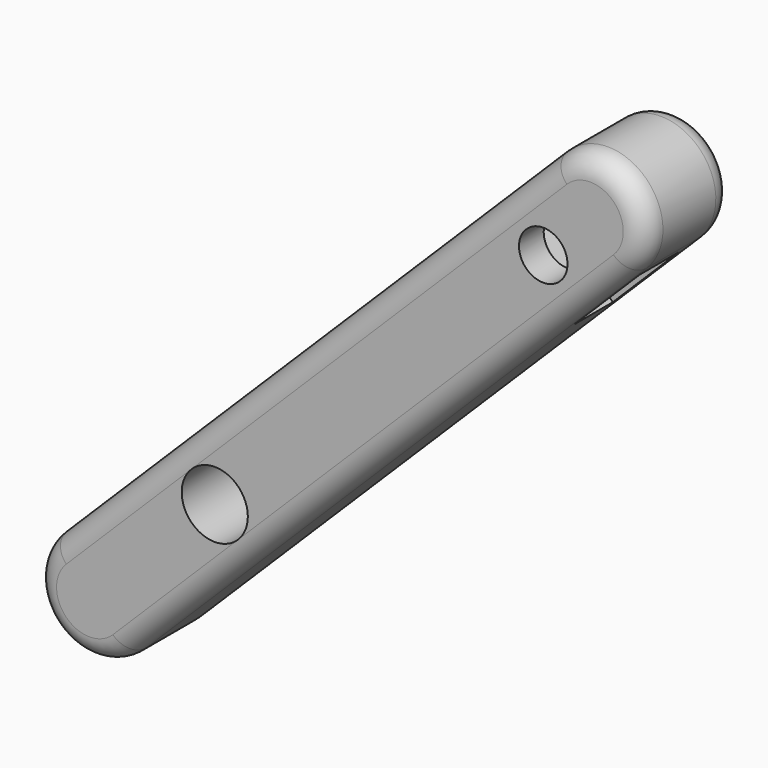
from build123d import *

# Parameters (mm, degrees)
F0_R     = 1.5
F1_DEPTH = 2.5
F2_DEPTH = 5
F3_R     = 0.99999
F6_DEPTH = 1.1
F7_D     = 2.2
F7_DEPTH = 2.501
F8_D     = 2.2


# Not quite as in the source:
# - a fillet or chamfer is up to 0.001 mm smaller than in the source, because OpenCascade refuses the exact size


with BuildPart() as f1:
    # F0 (on Front) → F1 (new body, symmetric)
    with BuildSketch(Plane.XZ):
        with BuildLine():
            ThreePointArc((-7.4377474476, -3.8639245472), (-7.4497190923, -7.3994381845), (-3.9142054549, -7.4114098292))
            Line((-3.9142054549, -7.4114098292), (18.78970035, 15.1392589236))
            ThreePointArc((18.78970035, 15.1392589236), (18.8016719947, 18.6747725609), (15.2661583574, 18.6867442056))
            Line((15.2661583574, 18.6867442056), (-7.4377474476, -3.8639245472))
        make_face()
        Circle(F0_R, mode=Mode.SUBTRACT)
        Circle(F0_R)
    extrude(amount=F1_DEPTH, both=True)

    # F0 (on Front) → F2 (cut, symmetric)
    with BuildSketch(Plane.XZ):
        Circle(F0_R)
    extrude(amount=F2_DEPTH, both=True, mode=Mode.SUBTRACT)

    # F3 (radius 1 in the source; OpenCascade refuses exactly that, so slightly less here)
    f3_edges = [f1.edges().sort_by_distance(p)[0] for p in [
        (3.914205, -2.5, 7.41141),
        (3.914205, 2.5, 7.41141),
    ]]
    fillet(f3_edges, radius=F3_R)

    # F5 (on Front) → F6 (cut, symmetric)
    with BuildSketch(Plane.XZ):
        Polygon((17.2437955285, 15.4185445413), (16.6082652356, 13.0784374397), (14.2639078916, 12.4587692675), (15.1712653624, 11.5452460911), (18.1511529993, 14.5050213649), align=None)
        Polygon((14.2639078916, 12.4587692675), (16.6082652356, 13.0784374397), (17.2437955285, 15.4185445413), (15.5349684774, 17.1389834706), (13.1906111334, 16.5193152984), (12.5550808405, 14.1792081968), align=None)
        Polygon((11.6477233698, 15.0927313731), (12.5550808405, 14.1792081968), (13.1906111334, 16.5193152984), (15.5349684774, 17.1389834706), (14.6276110067, 18.0525066469), align=None)
    extrude(amount=F6_DEPTH, both=True, mode=Mode.SUBTRACT)

    # F7 (through all, one way)
    with BuildSketch(Plane.XZ):
        with Locations((14.8994381845, 14.798876369)):
            Circle(F7_D / 2)
    extrude(amount=-F7_DEPTH, mode=Mode.SUBTRACT)

    # F8 (through all)
    with Locations(Plane(origin=(0, 0, 0), x_dir=(1, 0, 0), z_dir=(0, 1, 0))):
        with Locations((14.8994381845, -14.798876369)):
            Hole(F8_D / 2)


solid = f1.part
